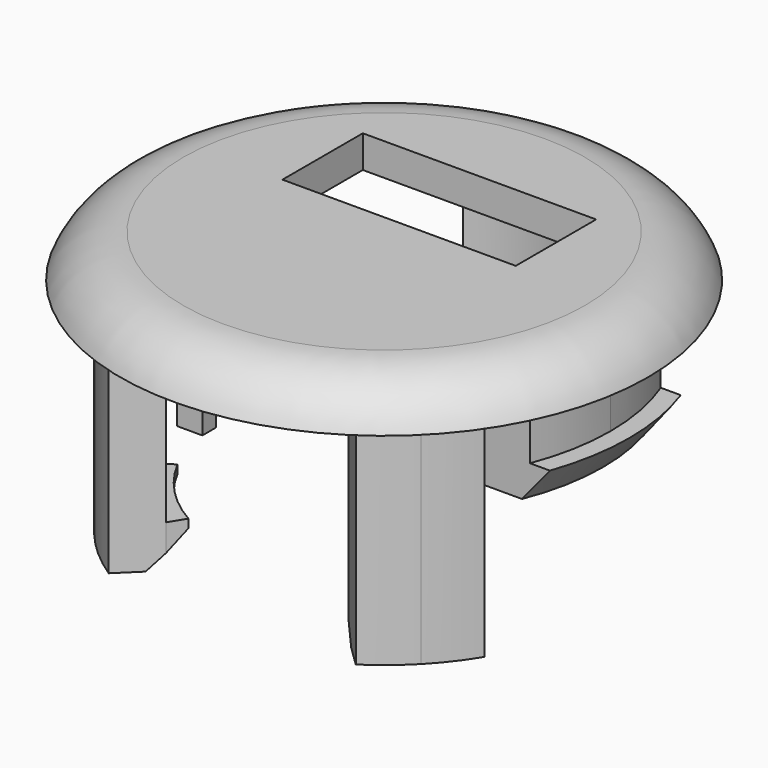
from build123d import *

# Parameters (mm, degrees)
F0_R          = 15.5
F1_DEPTH      = 2.5
F3_DEPTH      = 0.6
F4_DEPTH      = 2
F5_DEPTH      = 13
F6_DEPTH      = 10.5
F7_SIZE2      = 2
F7_SIZE       = 2
F8_DEPTH      = 5.5
F9_DEPTH      = 3.5
F10_T4_ANGLE  = 80.0083575427
F10_T9_ANGLE  = 80.0083575427
F10_T14_ANGLE = 69.1983444973
F10_S15_R     = 13.3
F10_T16_DEPTH = 10


# Not quite as in the source:
# - a fillet or chamfer that OpenCascade refuses, or shapes differently, is made with other operations: its cross-section is extruded or revolved along the edge and cut away or added
# - a feature names something its author has since deleted; it is built from what else it names


with BuildPart() as f1:
    # F0 (on Top) → F1 (new body)
    with BuildSketch(Plane.XY):
        Circle(F0_R)
        with BuildLine():
            ThreePointArc((3.5, 13.9681781203), (9.6909834568, 10.6510487578), (13.5764501988, 4.8))
            ThreePointArc((13.5764501988, 4.8), (14.192619259, 2.4350684937), (14.4, 0))
            ThreePointArc((14.4, 0), (14.192619259, -2.4350684937), (13.5764501988, -4.8))
            ThreePointArc((13.5764501988, -4.8), (0, -14.4), (-13.5764501988, -4.8))
            ThreePointArc((-13.5764501988, -4.8), (-14.4, 0), (-13.5764501988, 4.8))
            ThreePointArc((-13.5764501988, 4.8), (-9.6909834568, 10.6510487578), (-3.5, 13.9681781203))
            ThreePointArc((-3.5, 13.9681781203), (0, 14.4), (3.5, 13.9681781203))
        make_face(mode=Mode.SUBTRACT)
        with BuildLine():
            ThreePointArc((9.65, 0), (9.1363285843, 3.1064449134), (7.65, 5.8821764679))
            Line((7.65, 5.8821764679), (7.65, 0.2))
            Line((7.65, 0.2), (-7.65, 0.2))
            Line((-7.65, 0.2), (-7.65, 5.8821764679))
            ThreePointArc((-7.65, 5.8821764679), (-9.614696495, 0.8246886131), (-8.539960957, -4.4935027377))
            ThreePointArc((-8.539960957, -4.4935027377), (-7.8192632524, -5.6552296319), (-6.9416290733, -6.7034532749))
            Line((-6.9416290733, -6.7034532749), (0, 0))
            Line((0, 0), (6.9416290733, -6.7034532749))
            ThreePointArc((6.9416290733, -6.7034532749), (7.8192632524, -5.6552296319), (8.539960957, -4.4935027377))
            ThreePointArc((8.539960957, -4.4935027377), (9.3683809496, -2.3142900386), (9.65, 0))
        make_face()
        with BuildLine():
            ThreePointArc((4.7888057565, -8.3779376595), (5.9246729709, -7.6171353006), (6.9416290733, -6.7034532749))
            Line((6.9416290733, -6.7034532749), (0, 0))
            Line((0, 0), (-6.9416290733, -6.7034532749))
            ThreePointArc((-6.9416290733, -6.7034532749), (-5.9246729709, -7.6171353006), (-4.7888057565, -8.3779376595))
            ThreePointArc((-4.7888057565, -8.3779376595), (0, -9.65), (4.7888057565, -8.3779376595))
        make_face()
        with BuildLine():
            Line((13.5764501988, -4.8), (12.4036285014, -4.8))
            ThreePointArc((12.4036285014, -4.8), (11.9435522504, -5.8516288025), (11.3945125511, -6.8596708173))
            ThreePointArc((11.3945125511, -6.8596708173), (10.54816576, -8.1009998827), (9.5672193445, -9.2389563271))
            ThreePointArc((9.5672193445, -9.2389563271), (8.4641906486, -10.2590192837), (7.2531548444, -11.1481722629))
            ThreePointArc((7.2531548444, -11.1481722629), (4.1409605694, -12.6389258073), (0.75, -13.2788365454))
            Line((0.75, -13.2788365454), (0.75, -14.2788365454))
            Line((0.75, -14.2788365454), (-0.75, -14.2788365454))
            Line((-0.75, -14.2788365454), (-0.75, -13.2788365454))
            ThreePointArc((-0.75, -13.2788365454), (-4.1409605694, -12.6389258073), (-7.2531548444, -11.1481722629))
            ThreePointArc((-7.2531548444, -11.1481722629), (-8.4641906486, -10.2590192837), (-9.5672193445, -9.2389563271))
            ThreePointArc((-9.5672193445, -9.2389563271), (-10.54816576, -8.1009998827), (-11.3945125511, -6.8596708173))
            ThreePointArc((-11.3945125511, -6.8596708173), (-11.9435522504, -5.8516288025), (-12.4036285014, -4.8))
            Line((-12.4036285014, -4.8), (-13.5764501988, -4.8))
            ThreePointArc((-13.5764501988, -4.8), (0, -14.4), (13.5764501988, -4.8))
        make_face()
        with BuildLine():
            Line((7.2531548444, -11.1481722629), (5.3681959593, -9.3136980917))
            ThreePointArc((5.3681959593, -9.3136980917), (0, -10.75), (-5.3681959593, -9.3136980917))
            Line((-5.3681959593, -9.3136980917), (-7.2531548444, -11.1481722629))
            ThreePointArc((-7.2531548444, -11.1481722629), (-4.1409605694, -12.6389258073), (-0.75, -13.2788365454))
            ThreePointArc((-0.75, -13.2788365454), (0, -13.3), (0.75, -13.2788365454))
            ThreePointArc((0.75, -13.2788365454), (4.1409605694, -12.6389258073), (7.2531548444, -11.1481722629))
        make_face()
        with BuildLine():
            ThreePointArc((7.65, 7.5524830354), (8.7434224785, 6.2542036554), (9.618861679, 4.8))
            Line((9.618861679, 4.8), (12.4036285014, 4.8))
            ThreePointArc((12.4036285014, 4.8), (8.9082232352, 9.8759079984), (3.5, 12.8312119459))
            Line((3.5, 12.8312119459), (3.5, 10.1642756751))
            ThreePointArc((3.5, 10.1642756751), (5.512791423, 9.2288477464), (7.2905761089, 7.9))
            Line((7.2905761089, 7.9), (7.65, 7.9))
            Line((7.65, 7.9), (7.65, 7.5524830354))
        make_face()
        with BuildLine():
            Line((-3.5, 10.1642756751), (-3.5, 12.8312119459))
            ThreePointArc((-3.5, 12.8312119459), (-8.9082232352, 9.8759079984), (-12.4036285014, 4.8))
            Line((-12.4036285014, 4.8), (-9.618861679, 4.8))
            ThreePointArc((-9.618861679, 4.8), (-8.7434224785, 6.2542036554), (-7.65, 7.5524830354))
            Line((-7.65, 7.5524830354), (-7.65, 7.9))
            Line((-7.65, 7.9), (-7.2905761089, 7.9))
            ThreePointArc((-7.2905761089, 7.9), (-5.512791423, 9.2288477464), (-3.5, 10.1642756751))
        make_face()
        with BuildLine():
            ThreePointArc((9.618861679, 4.8), (10.4633948375, 2.4657389309), (10.75, 0))
            ThreePointArc((10.75, 0), (10.4633948375, -2.4657389309), (9.618861679, -4.8))
            Line((9.618861679, -4.8), (12.4036285014, -4.8))
            ThreePointArc((12.4036285014, -4.8), (13.0739867498, -2.441489395), (13.3, 0))
            ThreePointArc((13.3, 0), (13.0739867498, 2.441489395), (12.4036285014, 4.8))
            Line((12.4036285014, 4.8), (9.618861679, 4.8))
        make_face()
        with BuildLine():
            Line((-9.618861679, 4.8), (-12.4036285014, 4.8))
            ThreePointArc((-12.4036285014, 4.8), (-13.3, 0), (-12.4036285014, -4.8))
            Line((-12.4036285014, -4.8), (-9.618861679, -4.8))
            ThreePointArc((-9.618861679, -4.8), (-10.75, 0), (-9.618861679, 4.8))
        make_face()
        with BuildLine():
            Line((7.65, 0.2), (7.65, 5.8821764679))
            ThreePointArc((7.65, 5.8821764679), (7.2644168479, 6.3522238515), (6.85, 6.7970581872))
            Line((6.85, 6.7970581872), (6.85, 1.1))
            Line((6.85, 1.1), (-6.85, 1.1))
            Line((-6.85, 1.1), (-6.85, 6.7970581872))
            ThreePointArc((-6.85, 6.7970581872), (-7.2644168479, 6.3522238515), (-7.65, 5.8821764679))
            Line((-7.65, 5.8821764679), (-7.65, 0.2))
            Line((-7.65, 0.2), (7.65, 0.2))
        make_face()
        with BuildLine():
            Line((3.5, 10.1642756751), (3.5, 12.8312119459))
            ThreePointArc((3.5, 12.8312119459), (0, 13.3), (-3.5, 12.8312119459))
            Line((-3.5, 12.8312119459), (-3.5, 10.1642756751))
            ThreePointArc((-3.5, 10.1642756751), (0, 10.75), (3.5, 10.1642756751))
        make_face()
        with BuildLine():
            ThreePointArc((3.5, 12.8312119459), (8.9082232352, 9.8759079984), (12.4036285014, 4.8))
            Line((12.4036285014, 4.8), (13.5764501988, 4.8))
            ThreePointArc((13.5764501988, 4.8), (9.6909834568, 10.6510487578), (3.5, 13.9681781203))
            Line((3.5, 13.9681781203), (3.5, 12.8312119459))
        make_face()
        with BuildLine():
            ThreePointArc((-12.4036285014, 4.8), (-8.9082232352, 9.8759079984), (-3.5, 12.8312119459))
            Line((-3.5, 12.8312119459), (-3.5, 13.9681781203))
            ThreePointArc((-3.5, 13.9681781203), (-9.6909834568, 10.6510487578), (-13.5764501988, 4.8))
            Line((-13.5764501988, 4.8), (-12.4036285014, 4.8))
        make_face()
        with BuildLine():
            ThreePointArc((9.618861679, -4.8), (10.4633948375, -2.4657389309), (10.75, 0))
            ThreePointArc((10.75, 0), (10.4633948375, 2.4657389309), (9.618861679, 4.8))
            ThreePointArc((9.618861679, 4.8), (8.7434224785, 6.2542036554), (7.65, 7.5524830354))
            Line((7.65, 7.5524830354), (7.65, 5.8821764679))
            ThreePointArc((7.65, 5.8821764679), (9.1363285843, 3.1064449134), (9.65, 0))
            ThreePointArc((9.65, 0), (9.3683809496, -2.3142900386), (8.539960957, -4.4935027377))
            Line((8.539960957, -4.4935027377), (9.4953717756, -5.0398824235))
            ThreePointArc((9.4953717756, -5.0398824235), (9.557869325, -4.9203286441), (9.618861679, -4.8))
        make_face()
        with BuildLine():
            ThreePointArc((-8.539960957, -4.4935027377), (-9.614696495, 0.8246886131), (-7.65, 5.8821764679))
            Line((-7.65, 5.8821764679), (-7.65, 7.5524830354))
            ThreePointArc((-7.65, 7.5524830354), (-8.7434224785, 6.2542036554), (-9.618861679, 4.8))
            ThreePointArc((-9.618861679, 4.8), (-10.75, 0), (-9.618861679, -4.8))
            ThreePointArc((-9.618861679, -4.8), (-9.557869325, -4.9203286441), (-9.4953717756, -5.0398824235))
            Line((-9.4953717756, -5.0398824235), (-8.539960957, -4.4935027377))
        make_face()
        with BuildLine():
            Line((-5.5418859606, 7.9), (5.5418859606, 7.9))
            ThreePointArc((5.5418859606, 7.9), (4.1770435484, 8.6991268064), (2.7, 9.2645830991))
            ThreePointArc((2.7, 9.2645830991), (0, 9.65), (-2.7, 9.2645830991))
            ThreePointArc((-2.7, 9.2645830991), (-4.1770435484, 8.6991268064), (-5.5418859606, 7.9))
        make_face()
        with BuildLine():
            ThreePointArc((-5.3681959593, -9.3136980917), (0, -10.75), (5.3681959593, -9.3136980917))
            Line((5.3681959593, -9.3136980917), (4.7888057565, -8.3779376595))
            ThreePointArc((4.7888057565, -8.3779376595), (0, -9.65), (-4.7888057565, -8.3779376595))
            Line((-4.7888057565, -8.3779376595), (-5.3681959593, -9.3136980917))
        make_face()
        with BuildLine():
            ThreePointArc((6.6424769476, 7), (6.1087785088, 7.4702961876), (5.5418859606, 7.9))
            Line((5.5418859606, 7.9), (-5.5418859606, 7.9))
            ThreePointArc((-5.5418859606, 7.9), (-6.1087785088, 7.4702961876), (-6.6424769476, 7))
            Line((-6.6424769476, 7), (6.6424769476, 7))
        make_face()
        with BuildLine():
            ThreePointArc((-13.5764501988, 4.8), (-14.4, 0), (-13.5764501988, -4.8))
            Line((-13.5764501988, -4.8), (-12.4036285014, -4.8))
            ThreePointArc((-12.4036285014, -4.8), (-13.3, 0), (-12.4036285014, 4.8))
            Line((-12.4036285014, 4.8), (-13.5764501988, 4.8))
        make_face()
        with BuildLine():
            Line((13.5764501988, 4.8), (12.4036285014, 4.8))
            ThreePointArc((12.4036285014, 4.8), (13.0739867498, 2.441489395), (13.3, 0))
            ThreePointArc((13.3, 0), (13.0739867498, -2.441489395), (12.4036285014, -4.8))
            Line((12.4036285014, -4.8), (13.5764501988, -4.8))
            ThreePointArc((13.5764501988, -4.8), (14.192619259, -2.4350684937), (14.4, 0))
            ThreePointArc((14.4, 0), (14.192619259, 2.4350684937), (13.5764501988, 4.8))
        make_face()
        with BuildLine():
            ThreePointArc((-3.5, 12.8312119459), (0, 13.3), (3.5, 12.8312119459))
            Line((3.5, 12.8312119459), (3.5, 13.9681781203))
            ThreePointArc((3.5, 13.9681781203), (0, 14.4), (-3.5, 13.9681781203))
            Line((-3.5, 13.9681781203), (-3.5, 12.8312119459))
        make_face()
        with BuildLine():
            Line((11.3945125511, -6.8596708173), (9.4953717756, -5.0398824235))
            ThreePointArc((9.4953717756, -5.0398824235), (8.6992406278, -6.3155136371), (7.7329028536, -7.4675774824))
            Line((7.7329028536, -7.4675774824), (9.5672193445, -9.2389563271))
            ThreePointArc((9.5672193445, -9.2389563271), (10.54816576, -8.1009998827), (11.3945125511, -6.8596708173))
        make_face()
        with BuildLine():
            Line((9.5672193445, -9.2389563271), (7.7329028536, -7.4675774824))
            ThreePointArc((7.7329028536, -7.4675774824), (6.6152655164, -8.4735330381), (5.3681959593, -9.3136980917))
            Line((5.3681959593, -9.3136980917), (7.2531548444, -11.1481722629))
            ThreePointArc((7.2531548444, -11.1481722629), (8.4641906486, -10.2590192837), (9.5672193445, -9.2389563271))
        make_face()
        with BuildLine():
            Line((-7.2531548444, -11.1481722629), (-5.3681959593, -9.3136980917))
            ThreePointArc((-5.3681959593, -9.3136980917), (-6.6152655164, -8.4735330381), (-7.7329028536, -7.4675774824))
            Line((-7.7329028536, -7.4675774824), (-9.5672193445, -9.2389563271))
            ThreePointArc((-9.5672193445, -9.2389563271), (-8.4641906486, -10.2590192837), (-7.2531548444, -11.1481722629))
        make_face()
        with BuildLine():
            Line((-9.5672193445, -9.2389563271), (-7.7329028536, -7.4675774824))
            ThreePointArc((-7.7329028536, -7.4675774824), (-8.6992406278, -6.3155136371), (-9.4953717756, -5.0398824235))
            Line((-9.4953717756, -5.0398824235), (-11.3945125511, -6.8596708173))
            ThreePointArc((-11.3945125511, -6.8596708173), (-10.54816576, -8.1009998827), (-9.5672193445, -9.2389563271))
        make_face()
        with BuildLine():
            Line((2.7, 9.2645830991), (3.5, 10.1642756751))
            ThreePointArc((3.5, 10.1642756751), (0, 10.75), (-3.5, 10.1642756751))
            Line((-3.5, 10.1642756751), (-2.7, 9.2645830991))
            ThreePointArc((-2.7, 9.2645830991), (0, 9.65), (2.7, 9.2645830991))
        make_face()
        with BuildLine():
            Line((-2.7, 9.2645830991), (-3.5, 10.1642756751))
            ThreePointArc((-3.5, 10.1642756751), (-5.512791423, 9.2288477464), (-7.2905761089, 7.9))
            Line((-7.2905761089, 7.9), (-5.5418859606, 7.9))
            ThreePointArc((-5.5418859606, 7.9), (-4.1770435484, 8.6991268064), (-2.7, 9.2645830991))
        make_face()
        with BuildLine():
            Line((5.5418859606, 7.9), (7.2905761089, 7.9))
            ThreePointArc((7.2905761089, 7.9), (5.512791423, 9.2288477464), (3.5, 10.1642756751))
            Line((3.5, 10.1642756751), (2.7, 9.2645830991))
            ThreePointArc((2.7, 9.2645830991), (4.1770435484, 8.6991268064), (5.5418859606, 7.9))
        make_face()
        with BuildLine():
            Line((-9.618861679, -4.8), (-12.4036285014, -4.8))
            ThreePointArc((-12.4036285014, -4.8), (-11.9435522504, -5.8516288025), (-11.3945125511, -6.8596708173))
            Line((-11.3945125511, -6.8596708173), (-9.4953717756, -5.0398824235))
            ThreePointArc((-9.4953717756, -5.0398824235), (-9.557869325, -4.9203286441), (-9.618861679, -4.8))
        make_face()
        with BuildLine():
            Line((12.4036285014, -4.8), (9.618861679, -4.8))
            ThreePointArc((9.618861679, -4.8), (9.557869325, -4.9203286441), (9.4953717756, -5.0398824235))
            Line((9.4953717756, -5.0398824235), (11.3945125511, -6.8596708173))
            ThreePointArc((11.3945125511, -6.8596708173), (11.9435522504, -5.8516288025), (12.4036285014, -4.8))
        make_face()
        with BuildLine():
            ThreePointArc((5.3681959593, -9.3136980917), (6.6152655164, -8.4735330381), (7.7329028536, -7.4675774824))
            Line((7.7329028536, -7.4675774824), (6.9416290733, -6.7034532749))
            ThreePointArc((6.9416290733, -6.7034532749), (5.9246729709, -7.6171353006), (4.7888057565, -8.3779376595))
            Line((4.7888057565, -8.3779376595), (5.3681959593, -9.3136980917))
        make_face()
        with BuildLine():
            ThreePointArc((7.7329028536, -7.4675774824), (8.6992406278, -6.3155136371), (9.4953717756, -5.0398824235))
            Line((9.4953717756, -5.0398824235), (8.539960957, -4.4935027377))
            ThreePointArc((8.539960957, -4.4935027377), (7.8192632524, -5.6552296319), (6.9416290733, -6.7034532749))
            Line((6.9416290733, -6.7034532749), (7.7329028536, -7.4675774824))
        make_face()
        with BuildLine():
            ThreePointArc((-7.7329028536, -7.4675774824), (-6.6152655164, -8.4735330381), (-5.3681959593, -9.3136980917))
            Line((-5.3681959593, -9.3136980917), (-4.7888057565, -8.3779376595))
            ThreePointArc((-4.7888057565, -8.3779376595), (-5.9246729709, -7.6171353006), (-6.9416290733, -6.7034532749))
            Line((-6.9416290733, -6.7034532749), (-7.7329028536, -7.4675774824))
        make_face()
        with BuildLine():
            ThreePointArc((-9.4953717756, -5.0398824235), (-8.6992406278, -6.3155136371), (-7.7329028536, -7.4675774824))
            Line((-7.7329028536, -7.4675774824), (-6.9416290733, -6.7034532749))
            ThreePointArc((-6.9416290733, -6.7034532749), (-7.8192632524, -5.6552296319), (-8.539960957, -4.4935027377))
            Line((-8.539960957, -4.4935027377), (-9.4953717756, -5.0398824235))
        make_face()
        with BuildLine():
            ThreePointArc((-6.6424769476, 7), (-6.1087785088, 7.4702961876), (-5.5418859606, 7.9))
            Line((-5.5418859606, 7.9), (-7.2905761089, 7.9))
            ThreePointArc((-7.2905761089, 7.9), (-7.4723085875, 7.72833128), (-7.65, 7.5524830354))
            Line((-7.65, 7.5524830354), (-7.65, 5.8821764679))
            ThreePointArc((-7.65, 5.8821764679), (-7.2644168479, 6.3522238515), (-6.85, 6.7970581872))
            Line((-6.85, 6.7970581872), (-6.85, 7))
            Line((-6.85, 7), (-6.6424769476, 7))
        make_face()
        with BuildLine():
            Line((7.65, 5.8821764679), (7.65, 7.5524830354))
            ThreePointArc((7.65, 7.5524830354), (7.4723085875, 7.72833128), (7.2905761089, 7.9))
            Line((7.2905761089, 7.9), (5.5418859606, 7.9))
            ThreePointArc((5.5418859606, 7.9), (6.1087785088, 7.4702961876), (6.6424769476, 7))
            Line((6.6424769476, 7), (6.85, 7))
            Line((6.85, 7), (6.85, 6.7970581872))
            ThreePointArc((6.85, 6.7970581872), (7.2644168479, 6.3522238515), (7.65, 5.8821764679))
        make_face()
        with BuildLine():
            Line((0.75, -14.2788365454), (0.75, -13.2788365454))
            ThreePointArc((0.75, -13.2788365454), (0, -13.3), (-0.75, -13.2788365454))
            Line((-0.75, -13.2788365454), (-0.75, -14.2788365454))
            Line((-0.75, -14.2788365454), (0.75, -14.2788365454))
        make_face()
        with BuildLine():
            ThreePointArc((-7.65, 7.5524830354), (-7.4723085875, 7.72833128), (-7.2905761089, 7.9))
            Line((-7.2905761089, 7.9), (-7.65, 7.9))
            Line((-7.65, 7.9), (-7.65, 7.5524830354))
        make_face()
        with BuildLine():
            ThreePointArc((7.2905761089, 7.9), (7.4723085875, 7.72833128), (7.65, 7.5524830354))
            Line((7.65, 7.5524830354), (7.65, 7.9))
            Line((7.65, 7.9), (7.2905761089, 7.9))
        make_face()
    extrude(amount=F1_DEPTH)

    # F2: fillet of radius 4 on 1 edges, made by hand

    # F2_s1 → F2_t2 (revolve, cut)
    with BuildSketch(Plane.XZ):
        with BuildLine():
            ThreePointArc((15.5, 0), (14.027968734, 1.8166247904), (11.7919007565, 2.5))
            Line((11.7919007565, 2.5), (15.5, 2.5))
            Line((15.5, 2.5), (15.5, 0))
        make_face()
    revolve(axis=Axis((0, 0, 2.5), (0, 0, 1)), mode=Mode.SUBTRACT)

    # F0 (on Top) → F3 (cut)
    with BuildSketch(Plane.XY):
        with BuildLine():
            Line((7.65, 0.2), (7.65, 5.8821764679))
            ThreePointArc((7.65, 5.8821764679), (7.2644168479, 6.3522238515), (6.85, 6.7970581872))
            Line((6.85, 6.7970581872), (6.85, 1.1))
            Line((6.85, 1.1), (-6.85, 1.1))
            Line((-6.85, 1.1), (-6.85, 6.7970581872))
            ThreePointArc((-6.85, 6.7970581872), (-7.2644168479, 6.3522238515), (-7.65, 5.8821764679))
            Line((-7.65, 5.8821764679), (-7.65, 0.2))
            Line((-7.65, 0.2), (7.65, 0.2))
        make_face()
        with BuildLine():
            ThreePointArc((-6.6424769476, 7), (-6.1087785088, 7.4702961876), (-5.5418859606, 7.9))
            Line((-5.5418859606, 7.9), (-7.2905761089, 7.9))
            ThreePointArc((-7.2905761089, 7.9), (-7.4723085875, 7.72833128), (-7.65, 7.5524830354))
            Line((-7.65, 7.5524830354), (-7.65, 5.8821764679))
            ThreePointArc((-7.65, 5.8821764679), (-7.2644168479, 6.3522238515), (-6.85, 6.7970581872))
            Line((-6.85, 6.7970581872), (-6.85, 7))
            Line((-6.85, 7), (-6.6424769476, 7))
        make_face()
        with BuildLine():
            ThreePointArc((6.6424769476, 7), (6.1087785088, 7.4702961876), (5.5418859606, 7.9))
            Line((5.5418859606, 7.9), (-5.5418859606, 7.9))
            ThreePointArc((-5.5418859606, 7.9), (-6.1087785088, 7.4702961876), (-6.6424769476, 7))
            Line((-6.6424769476, 7), (6.6424769476, 7))
        make_face()
        with BuildLine():
            Line((7.65, 5.8821764679), (7.65, 7.5524830354))
            ThreePointArc((7.65, 7.5524830354), (7.4723085875, 7.72833128), (7.2905761089, 7.9))
            Line((7.2905761089, 7.9), (5.5418859606, 7.9))
            ThreePointArc((5.5418859606, 7.9), (6.1087785088, 7.4702961876), (6.6424769476, 7))
            Line((6.6424769476, 7), (6.85, 7))
            Line((6.85, 7), (6.85, 6.7970581872))
            ThreePointArc((6.85, 6.7970581872), (7.2644168479, 6.3522238515), (7.65, 5.8821764679))
        make_face()
        with BuildLine():
            ThreePointArc((7.2905761089, 7.9), (7.4723085875, 7.72833128), (7.65, 7.5524830354))
            Line((7.65, 7.5524830354), (7.65, 7.9))
            Line((7.65, 7.9), (7.2905761089, 7.9))
        make_face()
        with BuildLine():
            ThreePointArc((-7.65, 7.5524830354), (-7.4723085875, 7.72833128), (-7.2905761089, 7.9))
            Line((-7.2905761089, 7.9), (-7.65, 7.9))
            Line((-7.65, 7.9), (-7.65, 7.5524830354))
        make_face()
    extrude(amount=F3_DEPTH, mode=Mode.SUBTRACT)

    # F0 (on Top) → F4 (join)
    with BuildSketch(Plane.XY):
        with BuildLine():
            Line((0.75, -14.2788365454), (0.75, -13.2788365454))
            ThreePointArc((0.75, -13.2788365454), (0, -13.3), (-0.75, -13.2788365454))
            Line((-0.75, -13.2788365454), (-0.75, -14.2788365454))
            Line((-0.75, -14.2788365454), (0.75, -14.2788365454))
        make_face()
    extrude(amount=-F4_DEPTH)

    # F0 (on Top) → F5 (join)
    with BuildSketch(Plane.XY):
        with BuildLine():
            Line((-7.2531548444, -11.1481722629), (-5.3681959593, -9.3136980917))
            ThreePointArc((-5.3681959593, -9.3136980917), (-6.6152655164, -8.4735330381), (-7.7329028536, -7.4675774824))
            Line((-7.7329028536, -7.4675774824), (-9.5672193445, -9.2389563271))
            ThreePointArc((-9.5672193445, -9.2389563271), (-8.4641906486, -10.2590192837), (-7.2531548444, -11.1481722629))
        make_face()
        with BuildLine():
            Line((9.5672193445, -9.2389563271), (7.7329028536, -7.4675774824))
            ThreePointArc((7.7329028536, -7.4675774824), (6.6152655164, -8.4735330381), (5.3681959593, -9.3136980917))
            Line((5.3681959593, -9.3136980917), (7.2531548444, -11.1481722629))
            ThreePointArc((7.2531548444, -11.1481722629), (8.4641906486, -10.2590192837), (9.5672193445, -9.2389563271))
        make_face()
        with BuildLine():
            Line((11.3945125511, -6.8596708173), (9.4953717756, -5.0398824235))
            ThreePointArc((9.4953717756, -5.0398824235), (8.6992406278, -6.3155136371), (7.7329028536, -7.4675774824))
            Line((7.7329028536, -7.4675774824), (9.5672193445, -9.2389563271))
            ThreePointArc((9.5672193445, -9.2389563271), (10.54816576, -8.1009998827), (11.3945125511, -6.8596708173))
        make_face()
        with BuildLine():
            Line((3.5, 10.1642756751), (3.5, 12.8312119459))
            ThreePointArc((3.5, 12.8312119459), (0, 13.3), (-3.5, 12.8312119459))
            Line((-3.5, 12.8312119459), (-3.5, 10.1642756751))
            ThreePointArc((-3.5, 10.1642756751), (0, 10.75), (3.5, 10.1642756751))
        make_face()
        with BuildLine():
            Line((-9.5672193445, -9.2389563271), (-7.7329028536, -7.4675774824))
            ThreePointArc((-7.7329028536, -7.4675774824), (-8.6992406278, -6.3155136371), (-9.4953717756, -5.0398824235))
            Line((-9.4953717756, -5.0398824235), (-11.3945125511, -6.8596708173))
            ThreePointArc((-11.3945125511, -6.8596708173), (-10.54816576, -8.1009998827), (-9.5672193445, -9.2389563271))
        make_face()
        with BuildLine():
            Line((2.7, 9.2645830991), (3.5, 10.1642756751))
            ThreePointArc((3.5, 10.1642756751), (0, 10.75), (-3.5, 10.1642756751))
            Line((-3.5, 10.1642756751), (-2.7, 9.2645830991))
            ThreePointArc((-2.7, 9.2645830991), (0, 9.65), (2.7, 9.2645830991))
        make_face()
        with BuildLine():
            ThreePointArc((-9.4953717756, -5.0398824235), (-8.6992406278, -6.3155136371), (-7.7329028536, -7.4675774824))
            Line((-7.7329028536, -7.4675774824), (-6.9416290733, -6.7034532749))
            ThreePointArc((-6.9416290733, -6.7034532749), (-7.8192632524, -5.6552296319), (-8.539960957, -4.4935027377))
            Line((-8.539960957, -4.4935027377), (-9.4953717756, -5.0398824235))
        make_face()
        with BuildLine():
            ThreePointArc((-7.7329028536, -7.4675774824), (-6.6152655164, -8.4735330381), (-5.3681959593, -9.3136980917))
            Line((-5.3681959593, -9.3136980917), (-4.7888057565, -8.3779376595))
            ThreePointArc((-4.7888057565, -8.3779376595), (-5.9246729709, -7.6171353006), (-6.9416290733, -6.7034532749))
            Line((-6.9416290733, -6.7034532749), (-7.7329028536, -7.4675774824))
        make_face()
        with BuildLine():
            ThreePointArc((7.7329028536, -7.4675774824), (8.6992406278, -6.3155136371), (9.4953717756, -5.0398824235))
            Line((9.4953717756, -5.0398824235), (8.539960957, -4.4935027377))
            ThreePointArc((8.539960957, -4.4935027377), (7.8192632524, -5.6552296319), (6.9416290733, -6.7034532749))
            Line((6.9416290733, -6.7034532749), (7.7329028536, -7.4675774824))
        make_face()
        with BuildLine():
            ThreePointArc((5.3681959593, -9.3136980917), (6.6152655164, -8.4735330381), (7.7329028536, -7.4675774824))
            Line((7.7329028536, -7.4675774824), (6.9416290733, -6.7034532749))
            ThreePointArc((6.9416290733, -6.7034532749), (5.9246729709, -7.6171353006), (4.7888057565, -8.3779376595))
            Line((4.7888057565, -8.3779376595), (5.3681959593, -9.3136980917))
        make_face()
    extrude(amount=-F5_DEPTH)

    # F0 (on Top) → F6 (cut)
    with BuildSketch(Plane.XY):
        with BuildLine():
            ThreePointArc((5.3681959593, -9.3136980917), (6.6152655164, -8.4735330381), (7.7329028536, -7.4675774824))
            Line((7.7329028536, -7.4675774824), (6.9416290733, -6.7034532749))
            ThreePointArc((6.9416290733, -6.7034532749), (5.9246729709, -7.6171353006), (4.7888057565, -8.3779376595))
            Line((4.7888057565, -8.3779376595), (5.3681959593, -9.3136980917))
        make_face()
        with BuildLine():
            ThreePointArc((7.7329028536, -7.4675774824), (8.6992406278, -6.3155136371), (9.4953717756, -5.0398824235))
            Line((9.4953717756, -5.0398824235), (8.539960957, -4.4935027377))
            ThreePointArc((8.539960957, -4.4935027377), (7.8192632524, -5.6552296319), (6.9416290733, -6.7034532749))
            Line((6.9416290733, -6.7034532749), (7.7329028536, -7.4675774824))
        make_face()
        with BuildLine():
            Line((2.7, 9.2645830991), (3.5, 10.1642756751))
            ThreePointArc((3.5, 10.1642756751), (0, 10.75), (-3.5, 10.1642756751))
            Line((-3.5, 10.1642756751), (-2.7, 9.2645830991))
            ThreePointArc((-2.7, 9.2645830991), (0, 9.65), (2.7, 9.2645830991))
        make_face()
        with BuildLine():
            ThreePointArc((-7.7329028536, -7.4675774824), (-6.6152655164, -8.4735330381), (-5.3681959593, -9.3136980917))
            Line((-5.3681959593, -9.3136980917), (-4.7888057565, -8.3779376595))
            ThreePointArc((-4.7888057565, -8.3779376595), (-5.9246729709, -7.6171353006), (-6.9416290733, -6.7034532749))
            Line((-6.9416290733, -6.7034532749), (-7.7329028536, -7.4675774824))
        make_face()
        with BuildLine():
            ThreePointArc((-9.4953717756, -5.0398824235), (-8.6992406278, -6.3155136371), (-7.7329028536, -7.4675774824))
            Line((-7.7329028536, -7.4675774824), (-6.9416290733, -6.7034532749))
            ThreePointArc((-6.9416290733, -6.7034532749), (-7.8192632524, -5.6552296319), (-8.539960957, -4.4935027377))
            Line((-8.539960957, -4.4935027377), (-9.4953717756, -5.0398824235))
        make_face()
        with BuildLine():
            ThreePointArc((7.2905761089, 7.9), (7.4723085875, 7.72833128), (7.65, 7.5524830354))
            Line((7.65, 7.5524830354), (7.65, 7.9))
            Line((7.65, 7.9), (7.2905761089, 7.9))
        make_face()
    extrude(amount=-F6_DEPTH, mode=Mode.SUBTRACT)

    # F7
    f7_edges = [f1.edges().sort_by_distance(p)[0] for p in [
        (-6.941629, -6.703453, -13),
        (6.941629, -6.703453, -13),
        (0, 9.65, -13),
    ]]
    chamfer(f7_edges, length=F7_SIZE, length2=F7_SIZE2)

    # F0 (on Top) → F8 (join)
    with BuildSketch(Plane.XY):
        with BuildLine():
            ThreePointArc((9.618861679, 4.8), (10.4633948375, 2.4657389309), (10.75, 0))
            ThreePointArc((10.75, 0), (10.4633948375, -2.4657389309), (9.618861679, -4.8))
            Line((9.618861679, -4.8), (12.4036285014, -4.8))
            ThreePointArc((12.4036285014, -4.8), (13.0739867498, -2.441489395), (13.3, 0))
            ThreePointArc((13.3, 0), (13.0739867498, 2.441489395), (12.4036285014, 4.8))
            Line((12.4036285014, 4.8), (9.618861679, 4.8))
        make_face()
        with BuildLine():
            Line((13.5764501988, 4.8), (12.4036285014, 4.8))
            ThreePointArc((12.4036285014, 4.8), (13.0739867498, 2.441489395), (13.3, 0))
            ThreePointArc((13.3, 0), (13.0739867498, -2.441489395), (12.4036285014, -4.8))
            Line((12.4036285014, -4.8), (13.5764501988, -4.8))
            ThreePointArc((13.5764501988, -4.8), (14.192619259, -2.4350684937), (14.4, 0))
            ThreePointArc((14.4, 0), (14.192619259, 2.4350684937), (13.5764501988, 4.8))
        make_face()
        with BuildLine():
            ThreePointArc((-13.5764501988, 4.8), (-14.4, 0), (-13.5764501988, -4.8))
            Line((-13.5764501988, -4.8), (-12.4036285014, -4.8))
            ThreePointArc((-12.4036285014, -4.8), (-13.3, 0), (-12.4036285014, 4.8))
            Line((-12.4036285014, 4.8), (-13.5764501988, 4.8))
        make_face()
        with BuildLine():
            Line((-9.618861679, 4.8), (-12.4036285014, 4.8))
            ThreePointArc((-12.4036285014, 4.8), (-13.3, 0), (-12.4036285014, -4.8))
            Line((-12.4036285014, -4.8), (-9.618861679, -4.8))
            ThreePointArc((-9.618861679, -4.8), (-10.75, 0), (-9.618861679, 4.8))
        make_face()
        with BuildLine():
            ThreePointArc((-3.5, 12.8312119459), (0, 13.3), (3.5, 12.8312119459))
            Line((3.5, 12.8312119459), (3.5, 13.9681781203))
            ThreePointArc((3.5, 13.9681781203), (0, 14.4), (-3.5, 13.9681781203))
            Line((-3.5, 13.9681781203), (-3.5, 12.8312119459))
        make_face()
    extrude(amount=-F8_DEPTH)

    # F0 (on Top) → F9 (cut)
    with BuildSketch(Plane.XY):
        with BuildLine():
            Line((13.5764501988, 4.8), (12.4036285014, 4.8))
            ThreePointArc((12.4036285014, 4.8), (13.0739867498, 2.441489395), (13.3, 0))
            ThreePointArc((13.3, 0), (13.0739867498, -2.441489395), (12.4036285014, -4.8))
            Line((12.4036285014, -4.8), (13.5764501988, -4.8))
            ThreePointArc((13.5764501988, -4.8), (14.192619259, -2.4350684937), (14.4, 0))
            ThreePointArc((14.4, 0), (14.192619259, 2.4350684937), (13.5764501988, 4.8))
        make_face()
        with BuildLine():
            ThreePointArc((-13.5764501988, 4.8), (-14.4, 0), (-13.5764501988, -4.8))
            Line((-13.5764501988, -4.8), (-12.4036285014, -4.8))
            ThreePointArc((-12.4036285014, -4.8), (-13.3, 0), (-12.4036285014, 4.8))
            Line((-12.4036285014, 4.8), (-13.5764501988, 4.8))
        make_face()
        with BuildLine():
            ThreePointArc((-3.5, 12.8312119459), (0, 13.3), (3.5, 12.8312119459))
            Line((3.5, 12.8312119459), (3.5, 13.9681781203))
            ThreePointArc((3.5, 13.9681781203), (0, 14.4), (-3.5, 13.9681781203))
            Line((-3.5, 13.9681781203), (-3.5, 12.8312119459))
        make_face()
    extrude(amount=-F9_DEPTH, mode=Mode.SUBTRACT)

    # F10: chamfer of 2 x 1.534653976 on 3 edges, made by hand


with BuildPart() as f10_tool2:
    # F10_s3 → F10_t4 (revolve)
    with BuildSketch(Plane(origin=(0, 0, 0), x_dir=(0, 0, 1), z_dir=(-0.6428434781, -0.7659975604, 0))):
        Polygon((-5.5, -12.865346024), (-3.5, -14.4), (-5.5, -14.4), align=None)
    revolve(axis=Axis((0, 0, -5.5), (0, 0, 1)), revolution_arc=F10_T4_ANGLE)

    split(bisect_by=Plane.XZ.offset(4.8), keep=Keep.BOTTOM)


with BuildPart() as f1_1:
    add(f1.part)

    # F10_t1: cut F10_tool2
    add(f10_tool2.part, mode=Mode.SUBTRACT)


with BuildPart() as f10_tool7:
    # F10_s8 → F10_t9 (revolve)
    with BuildSketch(Plane(origin=(0, 0, 0), x_dir=(0, 0, 1), z_dir=(0.6428434781, 0.7659975604, 0))):
        Polygon((-5.5, -12.865346024), (-3.5, -14.4), (-5.5, -14.4), align=None)
    revolve(axis=Axis((0, 0, -5.5), (0, 0, 1)), revolution_arc=F10_T9_ANGLE)

    split(bisect_by=Plane.XZ.offset(4.8), keep=Keep.BOTTOM)


with BuildPart() as f1_2:
    add(f1_1.part)

    # F10_t6: cut F10_tool7
    add(f10_tool7.part, mode=Mode.SUBTRACT)


with BuildPart() as f10_tool12:
    # F10_s13 → F10_t14 (revolve)
    with BuildSketch(Plane(origin=(0, 0, 0), x_dir=(0, 0, 1), z_dir=(0.8231445721, -0.5678318532, 0))):
        Polygon((-3.5, -14.4), (-5.5, -12.865346024), (-5.5, -14.4), align=None)
    revolve(axis=Axis((0, 0, -5.5), (0, 0, 1)), revolution_arc=F10_T14_ANGLE)

    # F10_s15 → F10_t16 (cut, symmetric)
    with BuildSketch(Plane.XY.offset(-4.5)):
        Circle(F10_S15_R)
    extrude(amount=F10_T16_DEPTH, both=True, mode=Mode.SUBTRACT)


with BuildPart() as f1_3:
    add(f1_2.part)

    # F10_t11: cut F10_tool12
    add(f10_tool12.part, mode=Mode.SUBTRACT)


solid = f1_3.part
